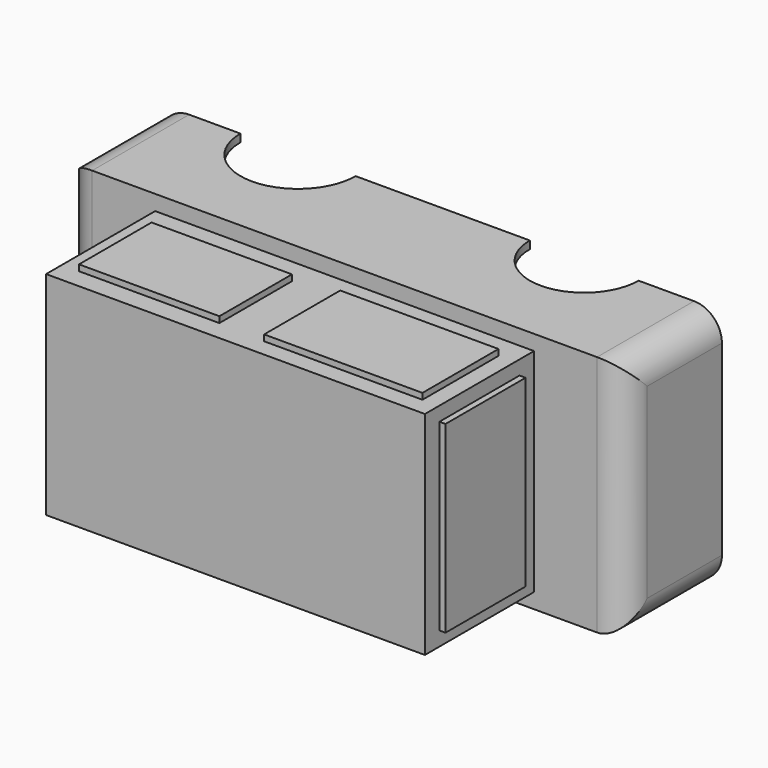
from build123d import *

# Parameters (mm, degrees)
F0_W        = 185
F0_H        = 80
F1_DEPTH    = 40
F2_W        = 125
F2_H        = 70
F3_DEPTH    = 45
F4_R        = 9.1981536726
F5_T        = 2.54
F5_T3_DEPTH = 130.08
F5_T5_DEPTH = 75.08
F7_DEPTH    = 112.6
F8_W        = 49.0510910749
F8_H        = 28.2043814659
F8_W_2      = 47.2116749734
F9_DEPTH    = 2
F10_W       = 52.2382371128
F10_H       = 31.3754677773
F10_W_2     = 46.3282726705
F10_H_2     = 29.9284607172
F11_DEPTH   = 2
F12_W       = 31.3480645418
F12_H       = 61.4709071815
F13_DEPTH   = 2
F14_W       = 33.0155193806
F14_H       = 60.6432519853
F15_DEPTH   = 2


# Not quite as in the source:
# - a shell that OpenCascade refuses in one call is made with other operations: the cavity is built on its own and cut out


with BuildPart() as f1:
    # F0 (on Front) → F1 (new body)
    with BuildSketch(Plane.XZ):
        Rectangle(F0_W, F0_H)
    extrude(amount=F1_DEPTH)

    # F2 (on face) → F3 (join)
    with BuildSketch(Plane.XZ.offset(40)):
        Rectangle(F2_W, F2_H)
    extrude(amount=F3_DEPTH)

    # F4
    f4_edges = [f1.edges().sort_by_distance(p)[0] for p in [
        (-92.5, -40, 0),
        (92.5, -40, 0),
        (92.5, -20, 40),
        (92.5, -20, -40),
        (-92.5, -20, -40),
        (-92.5, -20, 40),
    ]]
    fillet(f4_edges, radius=F4_R)

    # F5: shell of thickness 2.54, made by hand


with BuildPart() as f5_core1:
    # F5_t2: copy of F1
    add(f1.part)

    # the walls: a layer under each face that stays
    f5_faces = [f5_core1.faces().sort_by_distance(p)[0] for p in [
        (0, -20, 40),
        (89.8059231637, -20, 37.3059231637),
        (-89.8059231637, -20, 37.3059231637),
        (-71.4015825663, -40, -34.2857142857),
        (92.5, -15.4009231637, 0),
        (-92.5, -15.4009231637, 0),
        (89.8059231637, -20, -37.3059231637),
        (-89.8059231637, -20, -37.3059231637),
        (0, -20, -40),
        (89.8059231637, -37.3059231637, 0),
        (-89.8059231637, -37.3059231637, 0),
        (0, -62.5, 35),
        (-62.5, -62.5, 0),
        (0, -62.5, -35),
        (62.5, -62.5, 0),
        (0, -85, 0),
    ]]
    thicken(f5_faces, amount=-F5_T, mode=Mode.SUBTRACT)

    # F5_s4 → F5_t3 (cut)
    with BuildSketch(Plane.YZ.offset(-65.04)):
        Polygon((-40.0254, 35.0254), (-37.46, 35), (-37.46, 32.46), (-40, 32.46), align=None)
        Polygon((-40.0254, -35.0254), (-37.46, -35), (-37.46, -32.46), (-40, -32.46), align=None)
    extrude(amount=F5_T3_DEPTH, mode=Mode.SUBTRACT)

    # F5_s6 → F5_t5 (cut)
    with BuildSketch(Plane.XY.offset(-37.54)):
        Polygon((-62.5254, -40.0254), (-62.5, -37.46), (-59.96, -37.46), (-59.96, -40), align=None)
        Polygon((62.5254, -40.0254), (62.5, -37.46), (59.96, -37.46), (59.96, -40), align=None)
    extrude(amount=F5_T5_DEPTH, mode=Mode.SUBTRACT)


with BuildPart() as f1_1:
    add(f1.part)

    # what is left inside the walls is the cavity
    f5_cavity = [f5_core1.part.solids().sort_by_distance(p)[0] for p in [
        (0, -0.0254, -12.486667),
    ]]
    add(f5_cavity, mode=Mode.SUBTRACT)

    # F6 (on face) → F7 (cut)
    with BuildSketch(Plane.XY.offset(40)):
        with BuildLine():
            ThreePointArc((-66.3535060933, 0), (-47.3649650812, -18.9885410121), (-28.3764240691, 0))
            Line((-28.3764240691, 0), (-66.3535060933, 0))
        make_face()
        with BuildLine():
            Line((64.9945122235, 0), (29.1222798593, 0))
            ThreePointArc((29.1222798593, 0), (47.0583960414, -17.9361161821), (64.9945122235, 0))
        make_face()
    extrude(amount=-F7_DEPTH, mode=Mode.SUBTRACT)

    # F8 (on face) → F9 (join)
    with BuildSketch(Plane(origin=(0, 0, -35), x_dir=(1, 0, 0), z_dir=(0, 0, -1))):
        with Locations((-31.4233601093, 61.8686154485)):
            Rectangle(F8_W, F8_H)
        with Locations((32.0364944637, 61.8686154485)):
            Rectangle(F8_W_2, F8_H)
    extrude(amount=F9_DEPTH)

    # F10 (on face) → F11 (join)
    with BuildSketch(Plane.XY.offset(35)):
        with Locations((30.9228170663, -63.50582093)):
            Rectangle(F10_W, F10_H)
        with Locations((-33.6980968714, -63.50582093)):
            Rectangle(F10_W_2, F10_H_2)
    extrude(amount=F11_DEPTH)

    # F12 (on face) → F13 (join)
    with BuildSketch(Plane(origin=(-62.5, 0, 0), x_dir=(0, -1, 0), z_dir=(-1, 0, 0))):
        with Locations((62.5, 0)):
            Rectangle(F12_W, F12_H)
    extrude(amount=F13_DEPTH)

    # F14 (on face) → F15 (join)
    with BuildSketch(Plane.YZ.offset(62.5)):
        with Locations((-62.5, 0)):
            Rectangle(F14_W, F14_H)
    extrude(amount=F15_DEPTH)


solid = f1_1.part
